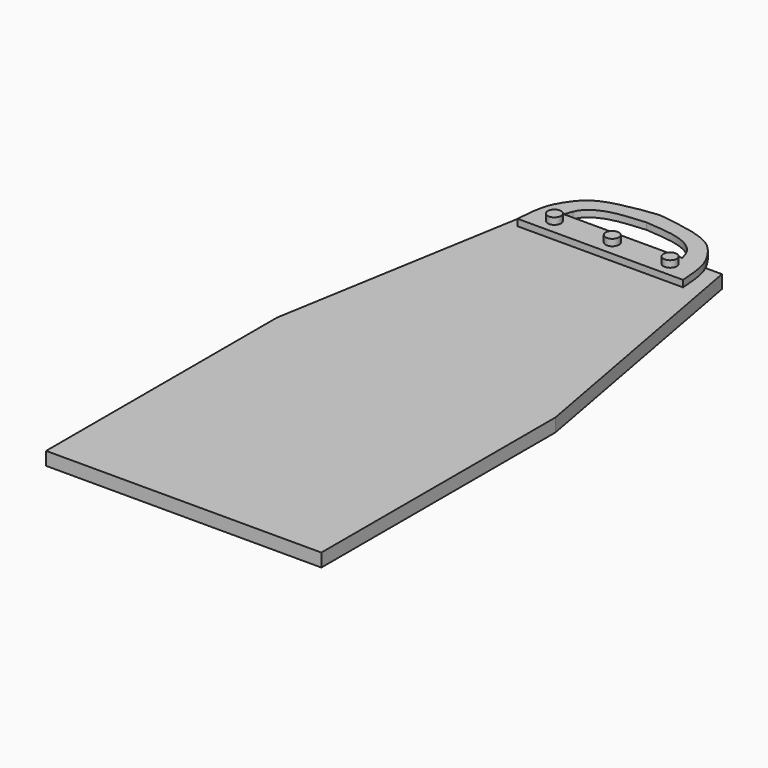
from build123d import *

# Parameters (mm, degrees)
F1_DEPTH = 1.27
F2_R     = 0.6409039012
F3_DEPTH = 1.27
F4_R     = 0.6409039012
F5_DEPTH = 0.635


with BuildPart() as f1:
    # F0 (on Top) → F1 (new body)
    with BuildSketch(Plane.XY):
        Polygon((4.5166932978, 54.1081428528), (0, 27.7454033494), (0, 0), (26.4549218118, 0), (26.4549218118, 28.1141139567), (21.6616950929, 54.1081428528), align=None)
    extrude(amount=F1_DEPTH)

    # F2 (on face) → F3 (join)
    with BuildSketch(Plane.XY.offset(1.27)):
        with Locations((7.2069587186, 52.051179111)):
            Circle(F2_R)
        with Locations((12.7762, 52.0446)):
            Circle(F2_R)
        with Locations((18.3454412814, 52.038020889)):
            Circle(F2_R)
    extrude(amount=F3_DEPTH)


with BuildPart() as f5:
    # F4 (on face) → F5 (new body)
    with BuildSketch(Plane.XY.offset(1.27)):
        with BuildLine():
            add(Edge.make_bspline(
                [(4.8227427374, 50.6045743823), (4.8876676433, 51.57466059), (4.9779603593, 52.8723637447), (5.3592032539, 53.8670811307), (5.4717375273, 54.1081428528)],
                knots=[0, 0, 0, 0, 0.1948044361, 0.262338147, 0.262338147, 0.262338147, 0.262338147], degree=3))
            Line((4.8227427374, 50.6045743823), (20.7296572626, 50.6045743823))
            add(Edge.make_bspline(
                [(20.7296572626, 50.6045743823), (20.6647323567, 51.57466059), (20.5744396407, 52.8723637447), (20.1931967461, 53.8670811307), (20.0806624727, 54.1081428528)],
                knots=[0, 0, 0, 0, 0.1948044361, 0.262338147, 0.262338147, 0.262338147, 0.262338147], degree=3))
            Line((20.0806624727, 54.1081428528), (18.2008306329, 54.1081428528))
            add(Edge.make_bspline(
                [(18.4601201523, 53.3456727862), (18.3838005475, 53.6044409864), (18.3074809427, 53.8632091865), (18.2008306329, 54.1081428528)],
                knots=[0, 0, 0, 0, 0.1299634207, 0.1299634207, 0.1299634207, 0.1299634207], degree=3))
            Line((18.4601201523, 53.3456727862), (12.7762, 53.3456727862))
            Line((12.7762, 53.3456727862), (7.0922798477, 53.3456727862))
            add(Edge.make_bspline(
                [(7.0922798477, 53.3456727862), (7.1685994525, 53.6044409864), (7.2449190573, 53.8632091865), (7.3515693671, 54.1081428528)],
                knots=[0, 0, 0, 0, 0.1299634207, 0.1299634207, 0.1299634207, 0.1299634207], degree=3))
            Line((7.3515693671, 54.1081428528), (5.4717375273, 54.1081428528))
        make_face()
        with Locations((7.2069587186, 52.051179111)):
            Circle(F4_R, mode=Mode.SUBTRACT)
        with Locations((12.7762, 52.0446)):
            Circle(F4_R, mode=Mode.SUBTRACT)
        with Locations((18.3454412814, 52.038020889)):
            Circle(F4_R, mode=Mode.SUBTRACT)
        with BuildLine():
            add(Edge.make_bspline(
                [(5.4717375273, 54.1081428528), (5.6289039905, 54.4448120036), (6.1137426448, 55.2493900595), (7.0873471955, 56.4104167137), (8.9314876501, 57.1332297998), (11.0322335818, 57.517239989), (12.2415750936, 57.6998275416), (12.7762, 57.738583535)],
                knots=[0.262338147, 0.262338147, 0.262338147, 0.262338147, 0.3566563861, 0.50920742, 0.6725861947, 0.8453952027, 1, 1, 1, 1], degree=3))
            Line((5.4717375273, 54.1081428528), (7.3515693671, 54.1081428528))
            add(Edge.make_bspline(
                [(7.3515693671, 54.1081428528), (7.4296103827, 54.2873722627), (7.7691891934, 54.9062304462), (9.0125467827, 55.7048152887), (10.8559336302, 56.0423099147), (12.1333636483, 56.1356138926), (12.7762, 56.182566906)],
                knots=[0.1299634207, 0.1299634207, 0.1299634207, 0.1299634207, 0.2250637291, 0.4724906838, 0.7345434509, 1, 1, 1, 1], degree=3))
            add(Edge.make_bspline(
                [(18.2008306329, 54.1081428528), (18.1227896173, 54.2873722627), (17.7832108066, 54.9062304462), (16.5398532173, 55.7048152887), (14.6964663698, 56.0423099147), (13.4190363517, 56.1356138926), (12.7762, 56.182566906)],
                knots=[0.1299634207, 0.1299634207, 0.1299634207, 0.1299634207, 0.2250637291, 0.4724906838, 0.7345434509, 1, 1, 1, 1], degree=3))
            Line((18.2008306329, 54.1081428528), (20.0806624727, 54.1081428528))
            add(Edge.make_bspline(
                [(20.0806624727, 54.1081428528), (19.9234960095, 54.4448120036), (19.4386573552, 55.2493900595), (18.4650528045, 56.4104167137), (16.6209123499, 57.1332297998), (14.5201664182, 57.517239989), (13.3108249064, 57.6998275416), (12.7762, 57.738583535)],
                knots=[0.262338147, 0.262338147, 0.262338147, 0.262338147, 0.3566563861, 0.50920742, 0.6725861947, 0.8453952027, 1, 1, 1, 1], degree=3))
        make_face()
    extrude(amount=F5_DEPTH)


solid = Compound([f1.part, f5.part])
